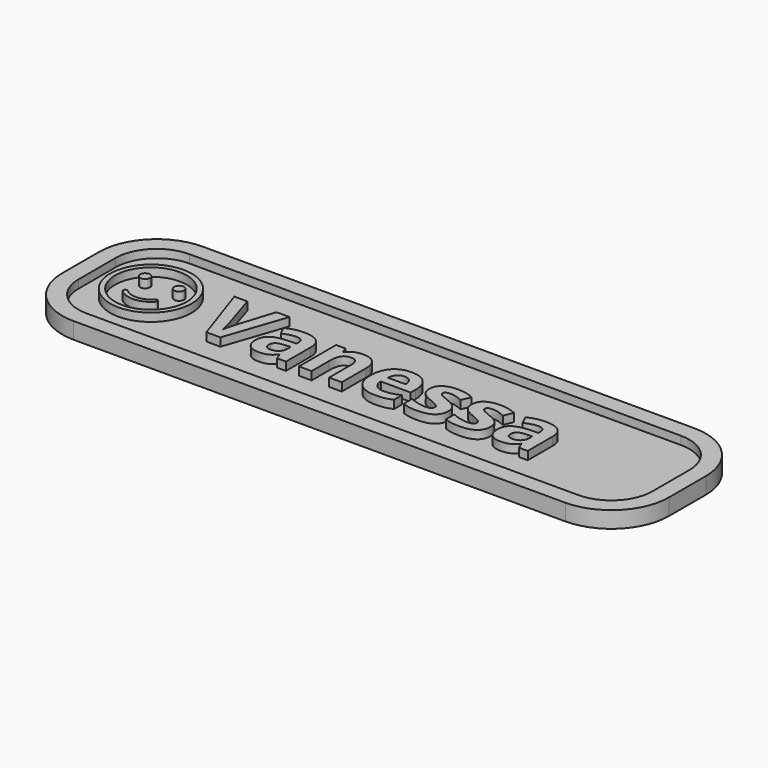
from build123d import *

# Parameters (mm, degrees)
F0_R         = 4.95
F0_R_2       = 4.35
F0_R_3       = 0.6
F0_TEXT_SIZE = 10.3268345507
F1_DEPTH     = 1
F2_DEPTH     = 2


# Not quite as in the source:
# - Text() gives the source's letters only with a copy of the font that has no kerning and outlines rounded to 1/6400 em; it was checked with that copy


with BuildPart() as f1:
    # F0 (on Top) → F1 (new body)
    with BuildSketch(Plane.XY):
        with BuildLine():
            ThreePointArc((36.8761118948, 2.8033320606), (34.8258593632, 7.7530795289), (29.8761118948, 9.8033320606))
            Line((29.8761118948, 9.8033320606), (-29.8761118948, 9.8033320606))
            ThreePointArc((-29.8761118948, 9.8033320606), (-34.8258593632, 7.7530795289), (-36.8761118948, 2.8033320606))
            Line((-36.8761118948, 2.8033320606), (-36.8761118948, -2.8033320606))
            ThreePointArc((-36.8761118948, -2.8033320606), (-34.8258593632, -7.7530795289), (-29.8761118948, -9.8033320606))
            Line((-29.8761118948, -9.8033320606), (29.8761118948, -9.8033320606))
            ThreePointArc((29.8761118948, -9.8033320606), (34.8258593632, -7.7530795289), (36.8761118948, -2.8033320606))
            Line((36.8761118948, -2.8033320606), (36.8761118948, 2.8033320606))
        make_face()
        with BuildLine():
            ThreePointArc((34.8761118948, -2.8033320606), (33.4116458008, -6.3388659665), (29.8761118948, -7.8033320606))
            Line((29.8761118948, -7.8033320606), (-29.8761118948, -7.8033320606))
            ThreePointArc((-29.8761118948, -7.8033320606), (-33.4116458008, -6.3388659665), (-34.8761118948, -2.8033320606))
            Line((-34.8761118948, -2.8033320606), (-34.8761118948, 2.8033320606))
            ThreePointArc((-34.8761118948, 2.8033320606), (-33.4116458008, 6.3388659665), (-29.8761118948, 7.8033320606))
            Line((-29.8761118948, 7.8033320606), (29.8761118948, 7.8033320606))
            ThreePointArc((29.8761118948, 7.8033320606), (33.4116458008, 6.3388659665), (34.8761118948, 2.8033320606))
            Line((34.8761118948, 2.8033320606), (34.8761118948, -2.8033320606))
        make_face(mode=Mode.SUBTRACT)
        with BuildLine():
            Line((-29.8761118948, -7.8033320606), (29.8761118948, -7.8033320606))
            ThreePointArc((29.8761118948, -7.8033320606), (33.4116458008, -6.3388659665), (34.8761118948, -2.8033320606))
            Line((34.8761118948, -2.8033320606), (34.8761118948, 2.8033320606))
            ThreePointArc((34.8761118948, 2.8033320606), (33.4116458008, 6.3388659665), (29.8761118948, 7.8033320606))
            Line((29.8761118948, 7.8033320606), (-29.8761118948, 7.8033320606))
            ThreePointArc((-29.8761118948, 7.8033320606), (-33.4116458008, 6.3388659665), (-34.8761118948, 2.8033320606))
            Line((-34.8761118948, 2.8033320606), (-34.8761118948, -2.8033320606))
            ThreePointArc((-34.8761118948, -2.8033320606), (-33.4116458008, -6.3388659665), (-29.8761118948, -7.8033320606))
        make_face()
        with Locations((-28.328852728, 0)):
            Circle(F0_R, mode=Mode.SUBTRACT)
        with BuildLine():
            Line((-17.3789330514, -0.7325598259), (-15.9831968191, 3.6547312902))
            Line((-15.9831968191, 3.6547312902), (-14.4051274143, 3.6547312902))
            Line((-14.4051274143, 3.6547312902), (-16.9109983608, -3.7176604383))
            Line((-16.9109983608, -3.7176604383), (-18.6149260617, -3.7176604383))
            Line((-18.6149260617, -3.7176604383), (-21.1159563044, 3.6547312902))
            Line((-21.1159563044, 3.6547312902), (-19.5378868996, 3.6547312902))
            Line((-19.5378868996, 3.6547312902), (-18.1502185069, -0.7325598259))
            add(Edge.make_bspline(
                [(-18.1502185069, -0.7325598259), (-18.0356551861, -1.1214296895), (-17.9114104579, -1.637771417)],
                knots=[0, 0, 0, 1, 1, 1], degree=2))
            add(Edge.make_bspline(
                [(-17.9114104579, -1.637771417), (-17.7871657297, -2.1541131446), (-17.7581215075, -2.3558091319)],
                knots=[0, 0, 0, 1, 1, 1], degree=2))
            add(Edge.make_bspline(
                [(-17.7581215075, -2.3558091319), (-17.7016466311, -1.892715145), (-17.3789330514, -0.7325598259)],
                knots=[0, 0, 0, 1, 1, 1], degree=2))
        make_face(mode=Mode.SUBTRACT)
        with BuildLine():
            Line((-8.9448136456, -3.7176604383), (-10.0178362982, -3.7176604383))
            Line((-10.0178362982, -3.7176604383), (-10.3163463594, -2.9512156865))
            Line((-10.3163463594, -2.9512156865), (-10.3566855569, -2.9512156865))
            add(Edge.make_bspline(
                [(-10.3566855569, -2.9512156865), (-10.7439418525, -3.4401267597), (-11.1554016667, -3.6297209878)],
                knots=[0, 0, 0, 1, 1, 1], degree=2))
            add(Edge.make_bspline(
                [(-11.1554016667, -3.6297209878), (-11.5668614808, -3.8193152159), (-12.2268107513, -3.8193152159)],
                knots=[0, 0, 0, 1, 1, 1], degree=2))
            add(Edge.make_bspline(
                [(-12.2268107513, -3.8193152159), (-13.0384354043, -3.8193152159), (-13.504756527, -3.3546076611)],
                knots=[0, 0, 0, 1, 1, 1], degree=2))
            add(Edge.make_bspline(
                [(-13.504756527, -3.3546076611), (-13.9710776496, -2.8899001063), (-13.9710776496, -2.0330955522)],
                knots=[0, 0, 0, 1, 1, 1], degree=2))
            add(Edge.make_bspline(
                [(-13.9710776496, -2.0330955522), (-13.9710776496, -1.1359518006), (-13.3433997371, -0.7099698754)],
                knots=[0, 0, 0, 1, 1, 1], degree=2))
            add(Edge.make_bspline(
                [(-13.3433997371, -0.7099698754), (-12.7157218246, -0.2839879501), (-11.4506845921, -0.238808049)],
                knots=[0, 0, 0, 1, 1, 1], degree=2))
            Line((-11.4506845921, -0.238808049), (-10.4712488777, -0.2081502589))
            Line((-10.4712488777, -0.2081502589), (-10.4712488777, 0.0387256296))
            add(Edge.make_bspline(
                [(-10.4712488777, 0.0387256296), (-10.4712488777, 0.8955301837), (-11.3490298145, 0.8955301837)],
                knots=[0, 0, 0, 1, 1, 1], degree=2))
            add(Edge.make_bspline(
                [(-11.3490298145, 0.8955301837), (-12.025114764, 0.8955301837), (-12.9383941946, 0.4872975054)],
                knots=[0, 0, 0, 1, 1, 1], degree=2))
            Line((-12.9383941946, 0.4872975054), (-13.4466680826, 1.526435232))
            add(Edge.make_bspline(
                [(-13.4466680826, 1.526435232), (-12.4736866398, 2.036322688), (-11.2893278022, 2.036322688)],
                knots=[0, 0, 0, 1, 1, 1], degree=2))
            add(Edge.make_bspline(
                [(-11.2893278022, 2.036322688), (-10.1549895696, 2.036322688), (-9.5499016076, 1.5417641271)],
                knots=[0, 0, 0, 1, 1, 1], degree=2))
            add(Edge.make_bspline(
                [(-9.5499016076, 1.5417641271), (-8.9448136456, 1.0472055662), (-8.9448136456, 0.0387256296)],
                knots=[0, 0, 0, 1, 1, 1], degree=2))
            Line((-8.9448136456, 0.0387256296), (-8.9448136456, -3.7176604383))
        make_face(mode=Mode.SUBTRACT)
        with BuildLine():
            Line((-2.1565334964, -0.0419527654), (-2.1565334964, -3.7176604383))
            Line((-2.1565334964, -3.7176604383), (-3.6942637037, -3.7176604383))
            Line((-3.6942637037, -3.7176604383), (-3.6942637037, -0.4243683573))
            add(Edge.make_bspline(
                [(-3.6942637037, -0.4243683573), (-3.6942637037, 0.1855603083), (-3.9112885861, 0.4905246412)],
                knots=[0, 0, 0, 1, 1, 1], degree=2))
            add(Edge.make_bspline(
                [(-3.9112885861, 0.4905246412), (-4.1283134685, 0.795488974), (-4.6027024306, 0.795488974)],
                knots=[0, 0, 0, 1, 1, 1], degree=2))
            add(Edge.make_bspline(
                [(-4.6027024306, 0.795488974), (-5.24812959, 0.795488974), (-5.535344676, 0.3646663451)],
                knots=[0, 0, 0, 1, 1, 1], degree=2))
            add(Edge.make_bspline(
                [(-5.535344676, 0.3646663451), (-5.8225597619, -0.0661562838), (-5.8225597619, -1.064954813)],
                knots=[0, 0, 0, 1, 1, 1], degree=2))
            Line((-5.8225597619, -1.064954813), (-5.8225597619, -3.7176604383))
            Line((-5.8225597619, -3.7176604383), (-7.3602899693, -3.7176604383))
            Line((-7.3602899693, -3.7176604383), (-7.3602899693, 1.9201457993))
            Line((-7.3602899693, 1.9201457993), (-6.1856125391, 1.9201457993))
            Line((-6.1856125391, 1.9201457993), (-5.9790758481, 1.1988809486))
            Line((-5.9790758481, 1.1988809486), (-5.8935567495, 1.1988809486))
            add(Edge.make_bspline(
                [(-5.8935567495, 1.1988809486), (-5.6353858857, 1.607113627), (-5.1843936581, 1.8160706698)],
                knots=[0, 0, 0, 1, 1, 1], degree=2))
            add(Edge.make_bspline(
                [(-5.1843936581, 1.8160706698), (-4.7334014304, 2.0250277127), (-4.1589712585, 2.0250277127)],
                knots=[0, 0, 0, 1, 1, 1], degree=2))
            add(Edge.make_bspline(
                [(-4.1589712585, 2.0250277127), (-3.1746948404, 2.0250277127), (-2.6656141684, 1.4933570901)],
                knots=[0, 0, 0, 1, 1, 1], degree=2))
            add(Edge.make_bspline(
                [(-2.6656141684, 1.4933570901), (-2.1565334964, 0.9616864675), (-2.1565334964, -0.0419527654)],
                knots=[0, 0, 0, 1, 1, 1], degree=2))
        make_face(mode=Mode.SUBTRACT)
        with BuildLine():
            add(Edge.make_bspline(
                [(3.0972435813, -3.7208875741), (2.6389902981, -3.8193152159), (1.9774274597, -3.8193152159)],
                knots=[0, 0, 0, 1, 1, 1], degree=2))
            add(Edge.make_bspline(
                [(1.9774274597, -3.8193152159), (0.6171897212, -3.8193152159), (-0.1492550306, -3.0673925752)],
                knots=[0, 0, 0, 1, 1, 1], degree=2))
            add(Edge.make_bspline(
                [(-0.1492550306, -3.0673925752), (-0.9156997824, -2.3154699344), (-0.9156997824, -0.939096517)],
                knots=[0, 0, 0, 1, 1, 1], degree=2))
            add(Edge.make_bspline(
                [(-0.9156997824, -0.939096517), (-0.9156997824, 0.477616098), (-0.207343475, 1.2513219053)],
                knots=[0, 0, 0, 1, 1, 1], degree=2))
            add(Edge.make_bspline(
                [(-0.207343475, 1.2513219053), (0.5010128325, 2.0250277127), (1.7515279539, 2.0250277127)],
                knots=[0, 0, 0, 1, 1, 1], degree=2))
            add(Edge.make_bspline(
                [(1.7515279539, 2.0250277127), (2.9455681988, 2.0250277127), (3.611164957, 1.3449088434)],
                knots=[0, 0, 0, 1, 1, 1], degree=2))
            add(Edge.make_bspline(
                [(3.611164957, 1.3449088434), (4.2767617151, 0.6647899742), (4.2767617151, -0.5357045423)],
                knots=[0, 0, 0, 1, 1, 1], degree=2))
            Line((4.2767617151, -0.5357045423), (4.2767617151, -1.2827864794))
            Line((4.2767617151, -1.2827864794), (0.6413932397, -1.2827864794))
            add(Edge.make_bspline(
                [(0.6413932397, -1.2827864794), (0.6672103261, -1.9378950462), (1.0302631032, -2.305788527)],
                knots=[0, 0, 0, 1, 1, 1], degree=2))
            add(Edge.make_bspline(
                [(1.0302631032, -2.305788527), (1.3933158804, -2.6736820079), (2.0484244472, -2.6736820079)],
                knots=[0, 0, 0, 1, 1, 1], degree=2))
            add(Edge.make_bspline(
                [(2.0484244472, -2.6736820079), (2.5583119032, -2.6736820079), (3.0117244827, -2.5679933105)],
                knots=[0, 0, 0, 1, 1, 1], degree=2))
            add(Edge.make_bspline(
                [(3.0117244827, -2.5679933105), (3.4651370621, -2.4623046132), (3.9588888391, -2.2299508358)],
                knots=[0, 0, 0, 1, 1, 1], degree=2))
            Line((3.9588888391, -2.2299508358), (3.9588888391, -3.4207639449))
            add(Edge.make_bspline(
                [(3.9588888391, -3.4207639449), (3.5554968645, -3.6224599323), (3.0972435813, -3.7208875741)],
                knots=[0, 0, 0, 1, 1, 1], degree=2))
        make_face(mode=Mode.SUBTRACT)
        with BuildLine():
            add(Edge.make_bspline(
                [(9.3143206944, -1.3223188929), (9.4611553732, -1.6248628738), (9.4611553732, -2.0427769596)],
                knots=[0, 0, 0, 1, 1, 1], degree=2))
            add(Edge.make_bspline(
                [(9.4611553732, -2.0427769596), (9.4611553732, -2.910876489), (8.8584877631, -3.3650958524)],
                knots=[0, 0, 0, 1, 1, 1], degree=2))
            add(Edge.make_bspline(
                [(8.8584877631, -3.3650958524), (8.255820153, -3.8193152159), (7.0553256364, -3.8193152159)],
                knots=[0, 0, 0, 1, 1, 1], degree=2))
            add(Edge.make_bspline(
                [(7.0553256364, -3.8193152159), (6.4405562671, -3.8193152159), (6.0065065024, -3.7354096852)],
                knots=[0, 0, 0, 1, 1, 1], degree=2))
            add(Edge.make_bspline(
                [(6.0065065024, -3.7354096852), (5.5724567377, -3.6515041544), (5.1948818494, -3.4901473646)],
                knots=[0, 0, 0, 1, 1, 1], degree=2))
            Line((5.1948818494, -3.4901473646), (5.1948818494, -2.2202694284))
            add(Edge.make_bspline(
                [(5.1948818494, -2.2202694284), (5.6224773425, -2.4219654157), (6.1597954527, -2.5583119032)],
                knots=[0, 0, 0, 1, 1, 1], degree=2))
            add(Edge.make_bspline(
                [(6.1597954527, -2.5583119032), (6.697113563, -2.6946583906), (7.1053462413, -2.6946583906)],
                knots=[0, 0, 0, 1, 1, 1], degree=2))
            add(Edge.make_bspline(
                [(7.1053462413, -2.6946583906), (7.9427879806, -2.6946583906), (7.9427879806, -2.210588021)],
                knots=[0, 0, 0, 1, 1, 1], degree=2))
            add(Edge.make_bspline(
                [(7.9427879806, -2.210588021), (7.9427879806, -2.0282548485), (7.8314517956, -1.9144983116)],
                knots=[0, 0, 0, 1, 1, 1], degree=2))
            add(Edge.make_bspline(
                [(7.8314517956, -1.9144983116), (7.7201156106, -1.8007417748), (7.4482294197, -1.6571342318)],
                knots=[0, 0, 0, 1, 1, 1], degree=2))
            add(Edge.make_bspline(
                [(7.4482294197, -1.6571342318), (7.1763432288, -1.5135266888), (6.7229306493, -1.3231256768)],
                knots=[0, 0, 0, 1, 1, 1], degree=2))
            add(Edge.make_bspline(
                [(6.7229306493, -1.3231256768), (6.0726627862, -1.050432702), (5.7668916694, -0.8180789246)],
                knots=[0, 0, 0, 1, 1, 1], degree=2))
            add(Edge.make_bspline(
                [(5.7668916694, -0.8180789246), (5.4611205527, -0.5857251472), (5.3231604973, -0.285601518)],
                knots=[0, 0, 0, 1, 1, 1], degree=2))
            add(Edge.make_bspline(
                [(5.3231604973, -0.285601518), (5.185200442, 0.0145221111), (5.185200442, 0.4517990116)],
                knots=[0, 0, 0, 1, 1, 1], degree=2))
            add(Edge.make_bspline(
                [(5.185200442, 0.4517990116), (5.185200442, 1.2037216523), (5.7668916694, 1.6143746825)],
                knots=[0, 0, 0, 1, 1, 1], degree=2))
            add(Edge.make_bspline(
                [(5.7668916694, 1.6143746825), (6.3485828969, 2.0250277127), (7.4183784136, 2.0250277127)],
                knots=[0, 0, 0, 1, 1, 1], degree=2))
            add(Edge.make_bspline(
                [(7.4183784136, 2.0250277127), (8.4365397576, 2.0250277127), (9.399839793, 1.5812965406)],
                knots=[0, 0, 0, 1, 1, 1], degree=2))
            Line((9.399839793, 1.5812965406), (8.9367458061, 0.4727753943))
            add(Edge.make_bspline(
                [(8.9367458061, 0.4727753943), (8.5123774488, 0.6534949989), (8.144483968, 0.7696718876)],
                knots=[0, 0, 0, 1, 1, 1], degree=2))
            add(Edge.make_bspline(
                [(8.144483968, 0.7696718876), (7.7765904871, 0.8858487763), (7.3925613272, 0.8858487763)],
                knots=[0, 0, 0, 1, 1, 1], degree=2))
            add(Edge.make_bspline(
                [(7.3925613272, 0.8858487763), (6.711635674, 0.8858487763), (6.711635674, 0.5179552954)],
                knots=[0, 0, 0, 1, 1, 1], degree=2))
            add(Edge.make_bspline(
                [(6.711635674, 0.5179552954), (6.711635674, 0.3114186044), (6.9310809082, 0.159743222)],
                knots=[0, 0, 0, 1, 1, 1], degree=2))
            add(Edge.make_bspline(
                [(6.9310809082, 0.159743222), (7.1505261424, 0.0080678395), (7.8927673758, -0.2888286538)],
                knots=[0, 0, 0, 1, 1, 1], degree=2))
            add(Edge.make_bspline(
                [(7.8927673758, -0.2888286538), (8.5527166463, -0.556680925), (8.860101331, -0.7882279184)],
                knots=[0, 0, 0, 1, 1, 1], degree=2))
            add(Edge.make_bspline(
                [(8.860101331, -0.7882279184), (9.1674860156, -1.0197749119), (9.3143206944, -1.3223188929)],
                knots=[0, 0, 0, 1, 1, 1], degree=2))
        make_face(mode=Mode.SUBTRACT)
        with BuildLine():
            add(Edge.make_bspline(
                [(14.4470801797, -1.3223188929), (14.5939148585, -1.6248628738), (14.5939148585, -2.0427769596)],
                knots=[0, 0, 0, 1, 1, 1], degree=2))
            add(Edge.make_bspline(
                [(14.5939148585, -2.0427769596), (14.5939148585, -2.910876489), (13.9912472484, -3.3650958524)],
                knots=[0, 0, 0, 1, 1, 1], degree=2))
            add(Edge.make_bspline(
                [(13.9912472484, -3.3650958524), (13.3885796383, -3.8193152159), (12.1880851217, -3.8193152159)],
                knots=[0, 0, 0, 1, 1, 1], degree=2))
            add(Edge.make_bspline(
                [(12.1880851217, -3.8193152159), (11.5733157524, -3.8193152159), (11.1392659877, -3.7354096852)],
                knots=[0, 0, 0, 1, 1, 1], degree=2))
            add(Edge.make_bspline(
                [(11.1392659877, -3.7354096852), (10.705216223, -3.6515041544), (10.3276413347, -3.4901473646)],
                knots=[0, 0, 0, 1, 1, 1], degree=2))
            Line((10.3276413347, -3.4901473646), (10.3276413347, -2.2202694284))
            add(Edge.make_bspline(
                [(10.3276413347, -2.2202694284), (10.7552368278, -2.4219654157), (11.292554938, -2.5583119032)],
                knots=[0, 0, 0, 1, 1, 1], degree=2))
            add(Edge.make_bspline(
                [(11.292554938, -2.5583119032), (11.8298730483, -2.6946583906), (12.2381057266, -2.6946583906)],
                knots=[0, 0, 0, 1, 1, 1], degree=2))
            add(Edge.make_bspline(
                [(12.2381057266, -2.6946583906), (13.0755474659, -2.6946583906), (13.0755474659, -2.210588021)],
                knots=[0, 0, 0, 1, 1, 1], degree=2))
            add(Edge.make_bspline(
                [(13.0755474659, -2.210588021), (13.0755474659, -2.0282548485), (12.9642112809, -1.9144983116)],
                knots=[0, 0, 0, 1, 1, 1], degree=2))
            add(Edge.make_bspline(
                [(12.9642112809, -1.9144983116), (12.8528750959, -1.8007417748), (12.580988905, -1.6571342318)],
                knots=[0, 0, 0, 1, 1, 1], degree=2))
            add(Edge.make_bspline(
                [(12.580988905, -1.6571342318), (12.3091027141, -1.5135266888), (11.8556901346, -1.3231256768)],
                knots=[0, 0, 0, 1, 1, 1], degree=2))
            add(Edge.make_bspline(
                [(11.8556901346, -1.3231256768), (11.2054222715, -1.050432702), (10.8996511547, -0.8180789246)],
                knots=[0, 0, 0, 1, 1, 1], degree=2))
            add(Edge.make_bspline(
                [(10.8996511547, -0.8180789246), (10.593880038, -0.5857251472), (10.4559199826, -0.285601518)],
                knots=[0, 0, 0, 1, 1, 1], degree=2))
            add(Edge.make_bspline(
                [(10.4559199826, -0.285601518), (10.3179599273, 0.0145221111), (10.3179599273, 0.4517990116)],
                knots=[0, 0, 0, 1, 1, 1], degree=2))
            add(Edge.make_bspline(
                [(10.3179599273, 0.4517990116), (10.3179599273, 1.2037216523), (10.8996511547, 1.6143746825)],
                knots=[0, 0, 0, 1, 1, 1], degree=2))
            add(Edge.make_bspline(
                [(10.8996511547, 1.6143746825), (11.4813423822, 2.0250277127), (12.5511378989, 2.0250277127)],
                knots=[0, 0, 0, 1, 1, 1], degree=2))
            add(Edge.make_bspline(
                [(12.5511378989, 2.0250277127), (13.5692992429, 2.0250277127), (14.5325992783, 1.5812965406)],
                knots=[0, 0, 0, 1, 1, 1], degree=2))
            Line((14.5325992783, 1.5812965406), (14.0695052914, 0.4727753943))
            add(Edge.make_bspline(
                [(14.0695052914, 0.4727753943), (13.6451369341, 0.6534949989), (13.2772434533, 0.7696718876)],
                knots=[0, 0, 0, 1, 1, 1], degree=2))
            add(Edge.make_bspline(
                [(13.2772434533, 0.7696718876), (12.9093499724, 0.8858487763), (12.5253208125, 0.8858487763)],
                knots=[0, 0, 0, 1, 1, 1], degree=2))
            add(Edge.make_bspline(
                [(12.5253208125, 0.8858487763), (11.8443951593, 0.8858487763), (11.8443951593, 0.5179552954)],
                knots=[0, 0, 0, 1, 1, 1], degree=2))
            add(Edge.make_bspline(
                [(11.8443951593, 0.5179552954), (11.8443951593, 0.3114186044), (12.0638403935, 0.159743222)],
                knots=[0, 0, 0, 1, 1, 1], degree=2))
            add(Edge.make_bspline(
                [(12.0638403935, 0.159743222), (12.2832856277, 0.0080678395), (13.0255268611, -0.2888286538)],
                knots=[0, 0, 0, 1, 1, 1], degree=2))
            add(Edge.make_bspline(
                [(13.0255268611, -0.2888286538), (13.6854761316, -0.556680925), (13.9928608163, -0.7882279184)],
                knots=[0, 0, 0, 1, 1, 1], degree=2))
            add(Edge.make_bspline(
                [(13.9928608163, -0.7882279184), (14.3002455009, -1.0197749119), (14.4470801797, -1.3223188929)],
                knots=[0, 0, 0, 1, 1, 1], degree=2))
        make_face(mode=Mode.SUBTRACT)
        with BuildLine():
            Line((20.4463256265, -3.7176604383), (19.373302974, -3.7176604383))
            Line((19.373302974, -3.7176604383), (19.0747929128, -2.9512156865))
            Line((19.0747929128, -2.9512156865), (19.0344537153, -2.9512156865))
            add(Edge.make_bspline(
                [(19.0344537153, -2.9512156865), (18.6471974196, -3.4401267597), (18.2357376055, -3.6297209878)],
                knots=[0, 0, 0, 1, 1, 1], degree=2))
            add(Edge.make_bspline(
                [(18.2357376055, -3.6297209878), (17.8242777914, -3.8193152159), (17.1643285209, -3.8193152159)],
                knots=[0, 0, 0, 1, 1, 1], degree=2))
            add(Edge.make_bspline(
                [(17.1643285209, -3.8193152159), (16.3527038679, -3.8193152159), (15.8863827452, -3.3546076611)],
                knots=[0, 0, 0, 1, 1, 1], degree=2))
            add(Edge.make_bspline(
                [(15.8863827452, -3.3546076611), (15.4200616225, -2.8899001063), (15.4200616225, -2.0330955522)],
                knots=[0, 0, 0, 1, 1, 1], degree=2))
            add(Edge.make_bspline(
                [(15.4200616225, -2.0330955522), (15.4200616225, -1.1359518006), (16.0477395351, -0.7099698754)],
                knots=[0, 0, 0, 1, 1, 1], degree=2))
            add(Edge.make_bspline(
                [(16.0477395351, -0.7099698754), (16.6754174476, -0.2839879501), (17.9404546801, -0.238808049)],
                knots=[0, 0, 0, 1, 1, 1], degree=2))
            Line((17.9404546801, -0.238808049), (18.9198903945, -0.2081502589))
            Line((18.9198903945, -0.2081502589), (18.9198903945, 0.0387256296))
            add(Edge.make_bspline(
                [(18.9198903945, 0.0387256296), (18.9198903945, 0.8955301837), (18.0421094577, 0.8955301837)],
                knots=[0, 0, 0, 1, 1, 1], degree=2))
            add(Edge.make_bspline(
                [(18.0421094577, 0.8955301837), (17.3660245082, 0.8955301837), (16.4527450776, 0.4872975054)],
                knots=[0, 0, 0, 1, 1, 1], degree=2))
            Line((16.4527450776, 0.4872975054), (15.9444711896, 1.526435232))
            add(Edge.make_bspline(
                [(15.9444711896, 1.526435232), (16.9174526324, 2.036322688), (18.1018114699, 2.036322688)],
                knots=[0, 0, 0, 1, 1, 1], degree=2))
            add(Edge.make_bspline(
                [(18.1018114699, 2.036322688), (19.2361497026, 2.036322688), (19.8412376646, 1.5417641271)],
                knots=[0, 0, 0, 1, 1, 1], degree=2))
            add(Edge.make_bspline(
                [(19.8412376646, 1.5417641271), (20.4463256265, 1.0472055662), (20.4463256265, 0.0387256296)],
                knots=[0, 0, 0, 1, 1, 1], degree=2))
            Line((20.4463256265, 0.0387256296), (20.4463256265, -3.7176604383))
        make_face(mode=Mode.SUBTRACT)
        with Locations((-28.328852728, 0)):
            Circle(F0_R)
        with Locations((-28.328852728, 0)):
            Circle(F0_R_2, mode=Mode.SUBTRACT)
        with Locations((-28.328852728, 0)):
            Circle(F0_R_2)
        with BuildLine():
            ThreePointArc((-29.7807970616, -1.7188244972), (-28.1667539551, -2.2441532897), (-26.6449624367, -1.4923181587))
            ThreePointArc((-26.6449624367, -1.4923181587), (-26.2920503867, -1.4710323662), (-26.2707645942, -1.8239444162))
            ThreePointArc((-26.2707645942, -1.8239444162), (-28.1307320056, -2.7428540208), (-30.1034513579, -2.1007854966))
            ThreePointArc((-30.1034513579, -2.1007854966), (-30.1331047094, -1.7484778487), (-29.7807970616, -1.7188244972))
        make_face(mode=Mode.SUBTRACT)
        with Locations((-30.3522536905, 1.6514693929)):
            Circle(F0_R_3, mode=Mode.SUBTRACT)
        with Locations((-26.2309277804, 1.6514693929)):
            Circle(F0_R_3, mode=Mode.SUBTRACT)
        with Locations((-21.1159563044, -3.7176604383)):
            Text('Vanessa', F0_TEXT_SIZE, font='Open Sans', font_style=FontStyle.BOLD, text_align=(TextAlign.LEFT, TextAlign.BOTTOM))
        with BuildLine():
            Line((18.9198903945, -1.5700015653), (18.9198903945, -1.1052940105))
            Line((18.9198903945, -1.1052940105), (18.3244838399, -1.1262703932))
            add(Edge.make_bspline(
                [(18.3244838399, -1.1262703932), (17.6532395941, -1.145633208), (17.3256853107, -1.367498794)],
                knots=[0, 0, 0, 1, 1, 1], degree=2))
            add(Edge.make_bspline(
                [(17.3256853107, -1.367498794), (16.9981310273, -1.5893643801), (16.9981310273, -2.0427769596)],
                knots=[0, 0, 0, 1, 1, 1], degree=2))
            add(Edge.make_bspline(
                [(16.9981310273, -2.0427769596), (16.9981310273, -2.6946583906), (17.7435993965, -2.6946583906)],
                knots=[0, 0, 0, 1, 1, 1], degree=2))
            add(Edge.make_bspline(
                [(17.7435993965, -2.6946583906), (18.2793039388, -2.6946583906), (18.5995971666, -2.386466922)],
                knots=[0, 0, 0, 1, 1, 1], degree=2))
            add(Edge.make_bspline(
                [(18.5995971666, -2.386466922), (18.9198903945, -2.0782754533), (18.9198903945, -1.5700015653)],
                knots=[0, 0, 0, 1, 1, 1], degree=2))
        make_face()
        with BuildLine():
            Line((-10.4712488777, -1.5700015653), (-10.4712488777, -1.1052940105))
            Line((-10.4712488777, -1.1052940105), (-11.0666554322, -1.1262703932))
            add(Edge.make_bspline(
                [(-11.0666554322, -1.1262703932), (-11.737899678, -1.145633208), (-12.0654539614, -1.367498794)],
                knots=[0, 0, 0, 1, 1, 1], degree=2))
            add(Edge.make_bspline(
                [(-12.0654539614, -1.367498794), (-12.3930082448, -1.5893643801), (-12.3930082448, -2.0427769596)],
                knots=[0, 0, 0, 1, 1, 1], degree=2))
            add(Edge.make_bspline(
                [(-12.3930082448, -2.0427769596), (-12.3930082448, -2.6946583906), (-11.6475398757, -2.6946583906)],
                knots=[0, 0, 0, 1, 1, 1], degree=2))
            add(Edge.make_bspline(
                [(-11.6475398757, -2.6946583906), (-11.1118353334, -2.6946583906), (-10.7915421055, -2.386466922)],
                knots=[0, 0, 0, 1, 1, 1], degree=2))
            add(Edge.make_bspline(
                [(-10.7915421055, -2.386466922), (-10.4712488777, -2.0782754533), (-10.4712488777, -1.5700015653)],
                knots=[0, 0, 0, 1, 1, 1], degree=2))
        make_face()
        with BuildLine():
            ThreePointArc((-26.2707645942, -1.8239444162), (-26.2920503867, -1.4710323662), (-26.6449624367, -1.4923181587))
            ThreePointArc((-26.6449624367, -1.4923181587), (-28.1667539551, -2.2441532897), (-29.7807970616, -1.7188244972))
            ThreePointArc((-29.7807970616, -1.7188244972), (-30.1331047094, -1.7484778487), (-30.1034513579, -2.1007854966))
            ThreePointArc((-30.1034513579, -2.1007854966), (-28.1307320056, -2.7428540208), (-26.2707645942, -1.8239444162))
        make_face()
        with BuildLine():
            add(Edge.make_bspline(
                [(2.5373355205, 0.6212236409), (2.2501204345, 0.9310286775), (1.7612093613, 0.9310286775)],
                knots=[0, 0, 0, 1, 1, 1], degree=2))
            add(Edge.make_bspline(
                [(1.7612093613, 0.9310286775), (1.272298288, 0.9310286775), (0.9947646095, 0.6212236409)],
                knots=[0, 0, 0, 1, 1, 1], degree=2))
            add(Edge.make_bspline(
                [(0.9947646095, 0.6212236409), (0.7172309309, 0.3114186044), (0.6768917334, -0.2581708638)],
                knots=[0, 0, 0, 1, 1, 1], degree=2))
            Line((0.6768917334, -0.2581708638), (2.8358455817, -0.2581708638))
            add(Edge.make_bspline(
                [(2.8358455817, -0.2581708638), (2.8245506064, 0.3114186044), (2.5373355205, 0.6212236409)],
                knots=[0, 0, 0, 1, 1, 1], degree=2))
        make_face()
        with Locations((-30.3522536905, 1.6514693929)):
            Circle(F0_R_3)
        with Locations((-26.2309277804, 1.6514693929)):
            Circle(F0_R_3)
    extrude(amount=F1_DEPTH)

    # F0 (on Top) → F2 (join)
    with BuildSketch(Plane.XY):
        with BuildLine():
            ThreePointArc((36.8761118948, 2.8033320606), (34.8258593632, 7.7530795289), (29.8761118948, 9.8033320606))
            Line((29.8761118948, 9.8033320606), (-29.8761118948, 9.8033320606))
            ThreePointArc((-29.8761118948, 9.8033320606), (-34.8258593632, 7.7530795289), (-36.8761118948, 2.8033320606))
            Line((-36.8761118948, 2.8033320606), (-36.8761118948, -2.8033320606))
            ThreePointArc((-36.8761118948, -2.8033320606), (-34.8258593632, -7.7530795289), (-29.8761118948, -9.8033320606))
            Line((-29.8761118948, -9.8033320606), (29.8761118948, -9.8033320606))
            ThreePointArc((29.8761118948, -9.8033320606), (34.8258593632, -7.7530795289), (36.8761118948, -2.8033320606))
            Line((36.8761118948, -2.8033320606), (36.8761118948, 2.8033320606))
        make_face()
        with BuildLine():
            ThreePointArc((34.8761118948, -2.8033320606), (33.4116458008, -6.3388659665), (29.8761118948, -7.8033320606))
            Line((29.8761118948, -7.8033320606), (-29.8761118948, -7.8033320606))
            ThreePointArc((-29.8761118948, -7.8033320606), (-33.4116458008, -6.3388659665), (-34.8761118948, -2.8033320606))
            Line((-34.8761118948, -2.8033320606), (-34.8761118948, 2.8033320606))
            ThreePointArc((-34.8761118948, 2.8033320606), (-33.4116458008, 6.3388659665), (-29.8761118948, 7.8033320606))
            Line((-29.8761118948, 7.8033320606), (29.8761118948, 7.8033320606))
            ThreePointArc((29.8761118948, 7.8033320606), (33.4116458008, 6.3388659665), (34.8761118948, 2.8033320606))
            Line((34.8761118948, 2.8033320606), (34.8761118948, -2.8033320606))
        make_face(mode=Mode.SUBTRACT)
        with Locations((-28.328852728, 0)):
            Circle(F0_R)
        with Locations((-28.328852728, 0)):
            Circle(F0_R_2, mode=Mode.SUBTRACT)
        with BuildLine():
            ThreePointArc((-26.2707645942, -1.8239444162), (-26.2920503867, -1.4710323662), (-26.6449624367, -1.4923181587))
            ThreePointArc((-26.6449624367, -1.4923181587), (-28.1667539551, -2.2441532897), (-29.7807970616, -1.7188244972))
            ThreePointArc((-29.7807970616, -1.7188244972), (-30.1331047094, -1.7484778487), (-30.1034513579, -2.1007854966))
            ThreePointArc((-30.1034513579, -2.1007854966), (-28.1307320056, -2.7428540208), (-26.2707645942, -1.8239444162))
        make_face()
        with Locations((-30.3522536905, 1.6514693929)):
            Circle(F0_R_3)
        with Locations((-26.2309277804, 1.6514693929)):
            Circle(F0_R_3)
        with Locations((-21.1159563044, -3.7176604383)):
            Text('Vanessa', F0_TEXT_SIZE, font='Open Sans', font_style=FontStyle.BOLD, text_align=(TextAlign.LEFT, TextAlign.BOTTOM))
    extrude(amount=F2_DEPTH)


solid = f1.part
